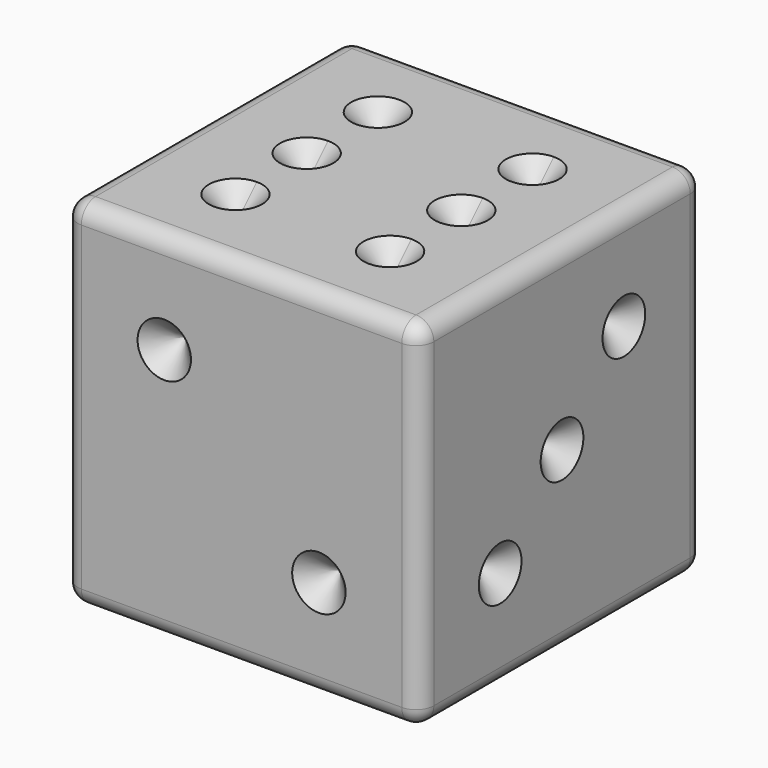
from build123d import *

# Parameters (mm, degrees)
F0_W      = 20
F0_H      = 20
F1_DEPTH  = 20
F2_R      = 1.5
F3_DEPTH  = 1.5
F4_R      = 1
F5_R      = 1.5
F6_DEPTH  = 1.5
F7_R      = 1.5
F8_DEPTH  = 1.5
F9_SIZE   = 1.49999
F10_SIZE  = 1.49999
F11_SIZE  = 1.49999
F12_R     = 1.5
F13_DEPTH = 1.5
F14_SIZE  = 1.49999
F15_R     = 1.5
F16_DEPTH = 1.5
F17_SIZE  = 1.49999
F19_DEPTH = 1.5
F20_SIZE  = 1.49999


# Not quite as in the source:
# - a fillet or chamfer is up to 0.001 mm smaller than in the source, because OpenCascade refuses the exact size


with BuildPart() as f1:
    # F0 (on Top) → F1 (new body)
    with BuildSketch(Plane.XY):
        with Locations((10, 10)):
            Rectangle(F0_W, F0_H)
    extrude(amount=F1_DEPTH)

    # F2 (on face) → F3 (cut)
    with BuildSketch(Plane.XZ):
        with Locations((5.6568542495, 14.3431457505)):
            Circle(F2_R)
        with Locations((14.3431457505, 5.6568542495)):
            Circle(F2_R)
    extrude(amount=-F3_DEPTH, mode=Mode.SUBTRACT)

    # F4
    f4_edges = [f1.edges().sort_by_distance(p)[0] for p in [
        (10, 0, 20),
        (20, 0, 10),
        (10, 0, 0),
        (0, 0, 10),
        (20, 10, 0),
        (10, 20, 0),
        (0, 10, 0),
        (20, 20, 10),
        (20, 10, 20),
        (10, 20, 20),
        (0, 10, 20),
        (0, 20, 10),
    ]]
    fillet(f4_edges, radius=F4_R)

    # F5 (on face) → F6 (cut)
    with BuildSketch(Plane.XY):
        with Locations((10, 10)):
            Circle(F5_R)
    extrude(amount=F6_DEPTH, mode=Mode.SUBTRACT)

    # F7 (on Right) → F8 (cut)
    with BuildSketch(Plane.YZ):
        with Locations((5.6568542495, 14.3431457505)):
            Circle(F7_R)
        with Locations((14.3431457505, 14.3431457505)):
            Circle(F7_R)
        with Locations((14.3431457505, 5.6568542495)):
            Circle(F7_R)
        with Locations((5.6568542495, 5.6568542495)):
            Circle(F7_R)
    extrude(amount=F8_DEPTH, mode=Mode.SUBTRACT)

    # F9 (size 1.5 in the source; OpenCascade refuses exactly that, so slightly less here)
    f9_edges = [f1.edges().sort_by_distance(p)[0] for p in [
        (4.156854, 1.5, 14.343146),
        (12.843146, 1.5, 5.656854),
    ]]
    chamfer(f9_edges, length=F9_SIZE)

    # F10 (size 1.5 in the source; OpenCascade refuses exactly that, so slightly less here)
    f10_edges = [f1.edges().sort_by_distance(p)[0] for p in [
        (1.5, 12.843146, 14.343146),
        (1.5, 4.156854, 14.343146),
        (1.5, 4.156854, 5.656854),
        (1.5, 12.843146, 5.656854),
    ]]
    chamfer(f10_edges, length=F10_SIZE)

    # F11 (size 1.5 in the source; OpenCascade refuses exactly that, so slightly less here)
    f11_edges = [f1.edges().sort_by_distance(p)[0] for p in [
        (8.5, 10, 1.5),
    ]]
    chamfer(f11_edges, length=F11_SIZE)

    # F12 (on face) → F13 (cut)
    with BuildSketch(Plane.YZ.offset(20)):
        with Locations((5.6568542495, 5.6568542495)):
            Circle(F12_R)
        with Locations((10, 10)):
            Circle(F12_R)
        with Locations((14.3431457505, 14.3431457505)):
            Circle(F12_R)
    extrude(amount=-F13_DEPTH, mode=Mode.SUBTRACT)

    # F14 (size 1.5 in the source; OpenCascade refuses exactly that, so slightly less here)
    f14_edges = [f1.edges().sort_by_distance(p)[0] for p in [
        (18.5, 8.5, 10),
        (18.5, 12.843146, 14.343146),
        (18.5, 4.156854, 5.656854),
    ]]
    chamfer(f14_edges, length=F14_SIZE)

    # F15 (on face) → F16 (cut)
    with BuildSketch(Plane(origin=(0, 20, 0), x_dir=(-1, 0, 0), z_dir=(0, 1, 0))):
        with Locations((-14.3431457505, 14.3431457505)):
            Circle(F15_R)
        with Locations((-5.6568542495, 5.6568542495)):
            Circle(F15_R)
        with Locations((-14.3431457505, 5.6568542495)):
            Circle(F15_R)
        with Locations((-5.6568542495, 14.3431457505)):
            Circle(F15_R)
        with Locations((-10, 10)):
            Circle(F15_R)
    extrude(amount=-F16_DEPTH, mode=Mode.SUBTRACT)

    # F17 (size 1.5 in the source; OpenCascade refuses exactly that, so slightly less here)
    f17_edges = [f1.edges().sort_by_distance(p)[0] for p in [
        (15.843146, 18.5, 14.343146),
        (7.156854, 18.5, 14.343146),
        (11.5, 18.5, 10),
        (15.843146, 18.5, 5.656854),
        (7.156854, 18.5, 5.656854),
    ]]
    chamfer(f17_edges, length=F17_SIZE)

    # F18 (on face) → F19 (cut)
    with BuildSketch(Plane.XY.offset(20)):
        with BuildLine():
            ThreePointArc((7.1568542495, 15), (4.5961940777, 16.0606601718), (5.6568542495, 13.5))
            ThreePointArc((5.6568542495, 13.5), (6.7175144213, 13.9393398282), (7.1568542495, 15))
        make_face()
        with BuildLine():
            ThreePointArc((5.6568542495, 11.5), (4.1568542495, 10), (5.6568542495, 8.5))
            Line((5.6568542495, 8.5), (5.6568542495, 10))
            Line((5.6568542495, 10), (5.6568542495, 11.5))
        make_face()
        with BuildLine():
            Line((5.6568542495, 10), (5.6568542495, 8.5))
            ThreePointArc((5.6568542495, 8.5), (6.7175144213, 8.9393398282), (7.1568542495, 10))
            ThreePointArc((7.1568542495, 10), (6.7175144213, 11.0606601718), (5.6568542495, 11.5))
            Line((5.6568542495, 11.5), (5.6568542495, 10))
        make_face()
        with BuildLine():
            ThreePointArc((5.6568542495, 6.5), (4.1568542495, 5), (5.6568542495, 3.5))
            Line((5.6568542495, 3.5), (5.6568542495, 5))
            Line((5.6568542495, 5), (5.6568542495, 6.5))
        make_face()
        with BuildLine():
            Line((5.6568542495, 5), (5.6568542495, 3.5))
            ThreePointArc((5.6568542495, 3.5), (6.7175144213, 3.9393398282), (7.1568542495, 5))
            ThreePointArc((7.1568542495, 5), (6.7175144213, 6.0606601718), (5.6568542495, 6.5))
            Line((5.6568542495, 6.5), (5.6568542495, 5))
        make_face()
        with BuildLine():
            ThreePointArc((14.3431457505, 16.5), (12.8431457505, 15), (14.3431457505, 13.5))
            Line((14.3431457505, 13.5), (14.3431457505, 15))
            Line((14.3431457505, 15), (14.3431457505, 16.5))
        make_face()
        with BuildLine():
            Line((14.3431457505, 15), (14.3431457505, 13.5))
            ThreePointArc((14.3431457505, 13.5), (15.4038059223, 13.9393398282), (15.8431457505, 15))
            ThreePointArc((15.8431457505, 15), (15.4038059223, 16.0606601718), (14.3431457505, 16.5))
            Line((14.3431457505, 16.5), (14.3431457505, 15))
        make_face()
        with BuildLine():
            ThreePointArc((14.3431457505, 11.5), (12.8431457505, 10), (14.3431457505, 8.5))
            Line((14.3431457505, 8.5), (14.3431457505, 10))
            Line((14.3431457505, 10), (14.3431457505, 11.5))
        make_face()
        with BuildLine():
            Line((14.3431457505, 10), (14.3431457505, 8.5))
            ThreePointArc((14.3431457505, 8.5), (15.4038059223, 8.9393398282), (15.8431457505, 10))
            ThreePointArc((15.8431457505, 10), (15.4038059223, 11.0606601718), (14.3431457505, 11.5))
            Line((14.3431457505, 11.5), (14.3431457505, 10))
        make_face()
        with BuildLine():
            ThreePointArc((14.3431457505, 6.5), (12.8431457505, 5), (14.3431457505, 3.5))
            Line((14.3431457505, 3.5), (14.3431457505, 5))
            Line((14.3431457505, 5), (14.3431457505, 6.5))
        make_face()
        with BuildLine():
            Line((14.3431457505, 5), (14.3431457505, 3.5))
            ThreePointArc((14.3431457505, 3.5), (15.4038059223, 3.9393398282), (15.8431457505, 5))
            ThreePointArc((15.8431457505, 5), (15.4038059223, 6.0606601718), (14.3431457505, 6.5))
            Line((14.3431457505, 6.5), (14.3431457505, 5))
        make_face()
    extrude(amount=-F19_DEPTH, mode=Mode.SUBTRACT)

    # F20 (size 1.5 in the source; OpenCascade refuses exactly that, so slightly less here)
    f20_edges = [f1.edges().sort_by_distance(p)[0] for p in [
        (5.656854, 6.5, 18.5),
        (5.656854, 11.5, 18.5),
        (5.656854, 16.5, 18.5),
        (14.343146, 16.5, 18.5),
        (14.343146, 6.5, 18.5),
        (14.343146, 11.5, 18.5),
    ]]
    chamfer(f20_edges, length=F20_SIZE)


solid = f1.part
